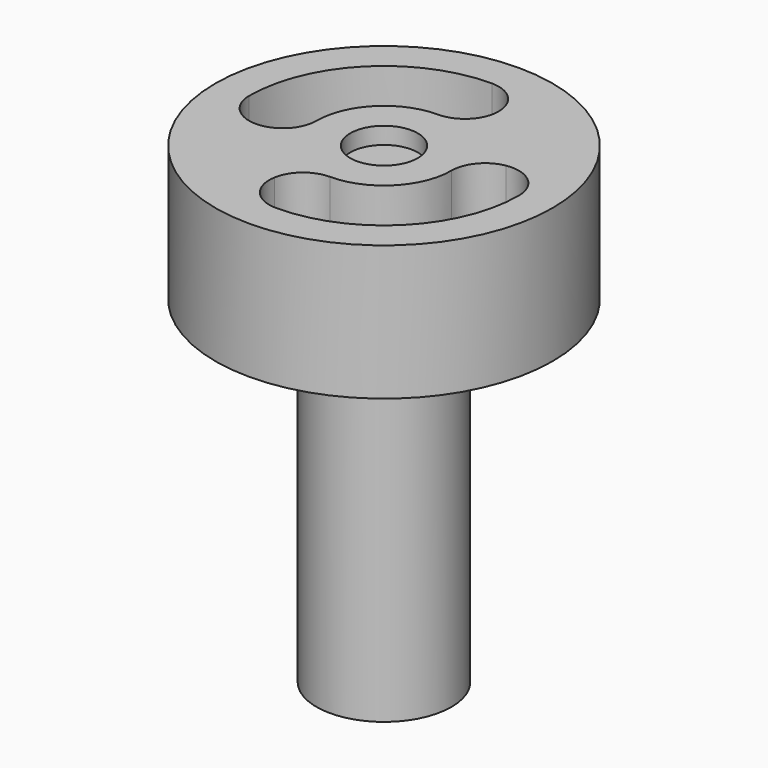
from build123d import *

# Parameters (mm, degrees)
F0_R     = 5
F0_R_2   = 1.5
F1_DEPTH = 2
F2_DEPTH = 2
F3_DEPTH = 2
F4_R     = 2
F4_R_2   = 1.5
F5_DEPTH = 10
F6_R     = 1
F7_DEPTH = 0.5


with BuildPart() as f1:
    # F0 (on Top) → F1 (new body)
    with BuildSketch(Plane.XY):
        with Locations((8, -12)):
            Circle(F0_R)
        with BuildLine():
            ThreePointArc((12, -12), (10.8284271247, -14.8284271247), (8, -16))
            ThreePointArc((8, -16), (7.2362373842, -15.6454972244), (7.0139867028, -14.8333333333))
            ThreePointArc((7.0139867028, -14.8333333333), (7.3545027756, -14.2362373842), (8, -14))
            ThreePointArc((8, -14), (9.4142135624, -13.4142135624), (10, -12))
            ThreePointArc((10, -12), (10.2362373842, -11.3545027756), (10.8333333333, -11.0139867028))
            ThreePointArc((10.8333333333, -11.0139867028), (11.6454972244, -11.2362373842), (12, -12))
        make_face(mode=Mode.SUBTRACT)
        with BuildLine():
            ThreePointArc((8, -10), (6.5857864376, -10.5857864376), (6, -12))
            ThreePointArc((6, -12), (5.7637626158, -12.6454972244), (5.1666666667, -12.9860132972))
            ThreePointArc((5.1666666667, -12.9860132972), (4.3545027756, -12.7637626158), (4, -12))
            ThreePointArc((4, -12), (5.1715728753, -9.1715728753), (8, -8))
            ThreePointArc((8, -8), (8.7071067812, -8.2928932188), (9, -9))
            ThreePointArc((9, -9), (8.9964971895, -9.0836262603), (8.9860132972, -9.1666666667))
            ThreePointArc((8.9860132972, -9.1666666667), (8.6454972244, -9.7637626158), (8, -10))
        make_face(mode=Mode.SUBTRACT)
        with Locations((8, -12)):
            Circle(F0_R_2, mode=Mode.SUBTRACT)
        with Locations((8, -12)):
            Circle(F0_R_2)
    extrude(amount=F1_DEPTH)

    # F0 (on Top) → F2 (join)
    with BuildSketch(Plane.XY):
        with Locations((8, -12)):
            Circle(F0_R)
        with BuildLine():
            ThreePointArc((12, -12), (10.8284271247, -14.8284271247), (8, -16))
            ThreePointArc((8, -16), (7.2362373842, -15.6454972244), (7.0139867028, -14.8333333333))
            ThreePointArc((7.0139867028, -14.8333333333), (7.3545027756, -14.2362373842), (8, -14))
            ThreePointArc((8, -14), (9.4142135624, -13.4142135624), (10, -12))
            ThreePointArc((10, -12), (10.2362373842, -11.3545027756), (10.8333333333, -11.0139867028))
            ThreePointArc((10.8333333333, -11.0139867028), (11.6454972244, -11.2362373842), (12, -12))
        make_face(mode=Mode.SUBTRACT)
        with BuildLine():
            ThreePointArc((8, -10), (6.5857864376, -10.5857864376), (6, -12))
            ThreePointArc((6, -12), (5.7637626158, -12.6454972244), (5.1666666667, -12.9860132972))
            ThreePointArc((5.1666666667, -12.9860132972), (4.3545027756, -12.7637626158), (4, -12))
            ThreePointArc((4, -12), (5.1715728753, -9.1715728753), (8, -8))
            ThreePointArc((8, -8), (8.7071067812, -8.2928932188), (9, -9))
            ThreePointArc((9, -9), (8.9964971895, -9.0836262603), (8.9860132972, -9.1666666667))
            ThreePointArc((8.9860132972, -9.1666666667), (8.6454972244, -9.7637626158), (8, -10))
        make_face(mode=Mode.SUBTRACT)
        with Locations((8, -12)):
            Circle(F0_R_2, mode=Mode.SUBTRACT)
        with BuildLine():
            ThreePointArc((9, -15), (8.7071067812, -15.7071067812), (8, -16))
            ThreePointArc((8, -16), (10.8284271247, -14.8284271247), (12, -12))
            ThreePointArc((12, -12), (11.6454972244, -12.7637626158), (10.8333333333, -12.9860132972))
            ThreePointArc((10.8333333333, -12.9860132972), (10.1213203436, -14.1213203436), (8.9860132972, -14.8333333333))
            ThreePointArc((8.9860132972, -14.8333333333), (8.9964971895, -14.9163737397), (9, -15))
        make_face()
        with BuildLine():
            ThreePointArc((8.9860132972, -14.8333333333), (10.1213203436, -14.1213203436), (10.8333333333, -12.9860132972))
            ThreePointArc((10.8333333333, -12.9860132972), (10.2362373842, -12.6454972244), (10, -12))
            ThreePointArc((10, -12), (9.4142135624, -13.4142135624), (8, -14))
            ThreePointArc((8, -14), (8.6454972244, -14.2362373842), (8.9860132972, -14.8333333333))
        make_face()
        with BuildLine():
            ThreePointArc((10.8333333333, -12.9860132972), (11.6454972244, -12.7637626158), (12, -12))
            ThreePointArc((12, -12), (11.6454972244, -11.2362373842), (10.8333333333, -11.0139867028))
            ThreePointArc((10.8333333333, -11.0139867028), (11, -12), (10.8333333333, -12.9860132972))
        make_face()
        with BuildLine():
            ThreePointArc((10.8333333333, -12.9860132972), (11, -12), (10.8333333333, -11.0139867028))
            ThreePointArc((10.8333333333, -11.0139867028), (10.2362373842, -11.3545027756), (10, -12))
            ThreePointArc((10, -12), (10.2362373842, -12.6454972244), (10.8333333333, -12.9860132972))
        make_face()
        with BuildLine():
            ThreePointArc((8, -14), (7.3545027756, -14.2362373842), (7.0139867028, -14.8333333333))
            ThreePointArc((7.0139867028, -14.8333333333), (8, -15), (8.9860132972, -14.8333333333))
            ThreePointArc((8.9860132972, -14.8333333333), (8.6454972244, -14.2362373842), (8, -14))
        make_face()
        with BuildLine():
            ThreePointArc((7.0139867028, -14.8333333333), (7.2362373842, -15.6454972244), (8, -16))
            ThreePointArc((8, -16), (8.7071067812, -15.7071067812), (9, -15))
            ThreePointArc((9, -15), (8.9964971895, -14.9163737397), (8.9860132972, -14.8333333333))
            ThreePointArc((8.9860132972, -14.8333333333), (8, -15), (7.0139867028, -14.8333333333))
        make_face()
        with BuildLine():
            ThreePointArc((7.0139867028, -9.1666666667), (7.3545027756, -9.7637626158), (8, -10))
            ThreePointArc((8, -10), (8.6454972244, -9.7637626158), (8.9860132972, -9.1666666667))
            ThreePointArc((8.9860132972, -9.1666666667), (8, -9), (7.0139867028, -9.1666666667))
        make_face()
        with BuildLine():
            ThreePointArc((8, -8), (7.2362373842, -8.3545027756), (7.0139867028, -9.1666666667))
            ThreePointArc((7.0139867028, -9.1666666667), (8, -9), (8.9860132972, -9.1666666667))
            ThreePointArc((8.9860132972, -9.1666666667), (8.9964971895, -9.0836262603), (9, -9))
            ThreePointArc((9, -9), (8.7071067812, -8.2928932188), (8, -8))
        make_face()
        with BuildLine():
            ThreePointArc((5.1666666667, -11.0139867028), (5.7637626158, -11.3545027756), (6, -12))
            ThreePointArc((6, -12), (6.5857864376, -10.5857864376), (8, -10))
            ThreePointArc((8, -10), (7.3545027756, -9.7637626158), (7.0139867028, -9.1666666667))
            ThreePointArc((7.0139867028, -9.1666666667), (7.2362373842, -8.3545027756), (8, -8))
            ThreePointArc((8, -8), (5.1715728753, -9.1715728753), (4, -12))
            ThreePointArc((4, -12), (4.3545027756, -11.2362373842), (5.1666666667, -11.0139867028))
        make_face()
        with BuildLine():
            ThreePointArc((5.1666666667, -12.9860132972), (5.7637626158, -12.6454972244), (6, -12))
            ThreePointArc((6, -12), (5.7637626158, -11.3545027756), (5.1666666667, -11.0139867028))
            ThreePointArc((5.1666666667, -11.0139867028), (5, -12), (5.1666666667, -12.9860132972))
        make_face()
        with BuildLine():
            ThreePointArc((5.1666666667, -12.9860132972), (5, -12), (5.1666666667, -11.0139867028))
            ThreePointArc((5.1666666667, -11.0139867028), (4.3545027756, -11.2362373842), (4, -12))
            ThreePointArc((4, -12), (4.3545027756, -12.7637626158), (5.1666666667, -12.9860132972))
        make_face()
    extrude(amount=-F2_DEPTH)

    # F0 (on Top) → F3 (join)
    with BuildSketch(Plane.XY):
        with Locations((8, -12)):
            Circle(F0_R_2)
    extrude(amount=-F3_DEPTH)

    # F4 (on face) → F5 (join)
    with BuildSketch(Plane(origin=(0, 0, -2), x_dir=(1, 0, 0), z_dir=(0, 0, -1))):
        with Locations((8, 12)):
            Circle(F4_R)
        with Locations((8, 12)):
            Circle(F4_R_2, mode=Mode.SUBTRACT)
        with Locations((8, 12)):
            Circle(F4_R_2)
    extrude(amount=F5_DEPTH)

    # F6 (on face) → F7 (cut)
    with BuildSketch(Plane.XY.offset(2)):
        with Locations((8, -12)):
            Circle(F6_R)
    extrude(amount=-F7_DEPTH, mode=Mode.SUBTRACT)


solid = f1.part
